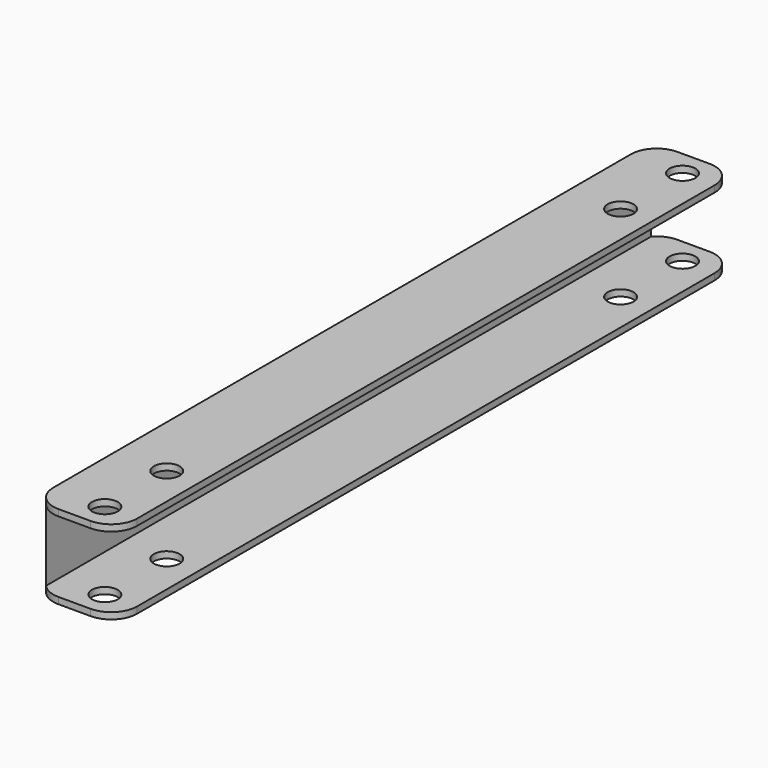
from build123d import *

# Parameters (mm, degrees)
F2_DEPTH    = 300
F1_R        = 5
F3_DEPTH    = 46
F4_T1_DEPTH = 52.5
F4_T3_DEPTH = 52.5
F4_T5_DEPTH = 82.5


# Not quite as in the source:
# - a fillet or chamfer that OpenCascade refuses, or shapes differently, is made with other operations: its cross-section is extruded or revolved along the edge and cut away or added
# - a pattern or mirror of a feature is missing from the dataset's text; its kind, count and spacing are read off the source's solid


with BuildPart() as f2:
    # F0 (on Front) → F2 (new body)
    with BuildSketch(Plane.XZ):
        Polygon((-74.9858543277, 32.5), (-74.9858543277, 0), (-42.4858543277, 0), (-42.4858543277, 2.5), (-72.4858543277, 2.5), (-72.4858543277, 30), (-42.4858543277, 30), (-42.4858543277, 32.5), align=None)
    extrude(amount=F2_DEPTH)

    # F1 (on Top) → F3 (cut)
    with BuildSketch(Plane.XY):
        with Locations((-54.9858543277, -260)):
            Circle(F1_R)
        with Locations((-54.9858543277, -40)):
            Circle(F1_R)
        with Locations((-54.9858543277, -10)):
            Circle(F1_R)
    f3 = extrude(amount=F3_DEPTH, mode=Mode.SUBTRACT)

    # F3_copies: F3 across plane
    add(f3.mirror(Plane(origin=(0, -275, 0), x_dir=(0, 0, -1), z_dir=(0, -1, 0))), mode=Mode.SUBTRACT)

    # F4: fillet of radius 10 on 6 edges, made by hand

    # F4_s2 → F4_t1 (cut)
    with BuildSketch(Plane.XY.offset(-25)):
        with BuildLine():
            ThreePointArc((-52.4858543277, 0), (-45.4147865158, -2.9289321881), (-42.4858543277, -10))
            Line((-42.4858543277, -10), (-42.4858543277, 0))
            Line((-42.4858543277, 0), (-52.4858543277, 0))
        make_face()
        with BuildLine():
            ThreePointArc((-52.4858543277, -300), (-45.4147865158, -297.0710678119), (-42.4858543277, -290))
            Line((-42.4858543277, -290), (-42.4858543277, -300))
            Line((-42.4858543277, -300), (-52.4858543277, -300))
        make_face()
    extrude(amount=F4_T1_DEPTH, mode=Mode.SUBTRACT)

    # F4_s4 → F4_t3 (cut)
    with BuildSketch(Plane.XY.offset(5)):
        with BuildLine():
            ThreePointArc((-42.4858543277, -10), (-45.4147865158, -2.9289321881), (-52.4858543277, 0))
            Line((-52.4858543277, 0), (-42.4858543277, 0))
            Line((-42.4858543277, 0), (-42.4858543277, -10))
        make_face()
        with BuildLine():
            ThreePointArc((-42.4858543277, -290), (-45.4147865158, -297.0710678119), (-52.4858543277, -300))
            Line((-52.4858543277, -300), (-42.4858543277, -300))
            Line((-42.4858543277, -300), (-42.4858543277, -290))
        make_face()
    extrude(amount=F4_T3_DEPTH, mode=Mode.SUBTRACT)

    # F4_s6 → F4_t5 (cut)
    with BuildSketch(Plane.XY.offset(-25)):
        with BuildLine():
            ThreePointArc((-64.9858543277, 0), (-72.0569221395, -2.9289321881), (-74.9858543277, -10))
            Line((-74.9858543277, -10), (-74.9858543277, 0))
            Line((-74.9858543277, 0), (-64.9858543277, 0))
        make_face()
        with BuildLine():
            ThreePointArc((-64.9858543277, -300), (-72.0569221395, -297.0710678119), (-74.9858543277, -290))
            Line((-74.9858543277, -290), (-74.9858543277, -300))
            Line((-74.9858543277, -300), (-64.9858543277, -300))
        make_face()
    extrude(amount=F4_T5_DEPTH, mode=Mode.SUBTRACT)


solid = f2.part
